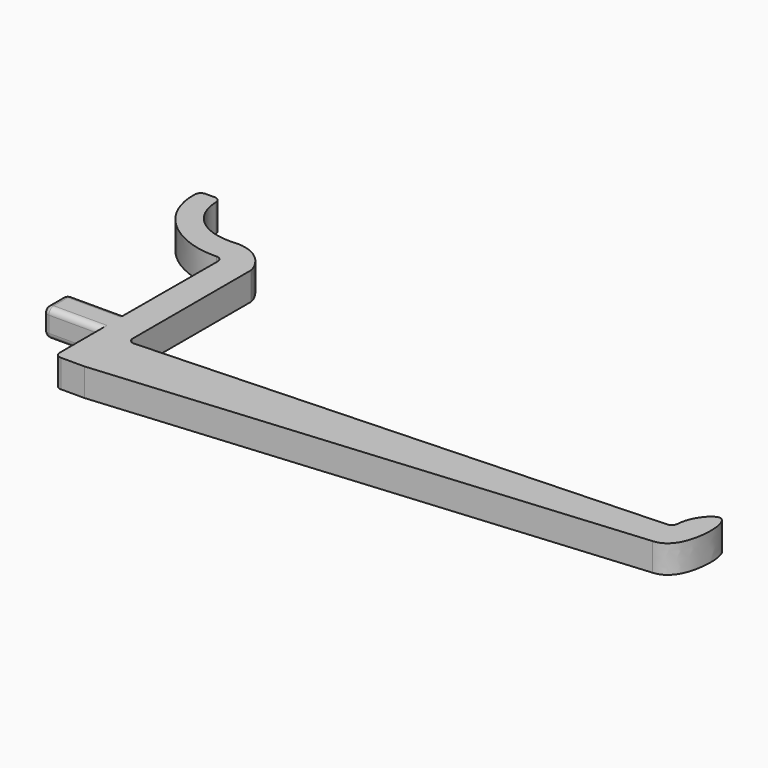
from build123d import *

# Parameters (mm, degrees)
F1_DEPTH = 4.7
F2_R     = 1


with BuildPart() as f1:
    # F0 (on Top) → F1 (new body)
    with BuildSketch(Plane.XY):
        with BuildLine():
            Line((-12.3301572212, 26.1715785798), (-15.8301572212, 26.1715785798))
            add(Edge.make_bspline(
                [(-15.8301572212, 26.1715785798), (-16.7997692679, 17.9848263993), (-8.8800950357, 12.3493980705), (-1.5833711872, 13.1881022432)],
                knots=[0, 0, 0, 0, 19.2754136163, 19.2754136163, 19.2754136163, 19.2754136163], degree=3))
            Line((-1.5833711872, 13.1881022432), (-1.6532300643, -7.3117787256))
            Line((-1.6532300643, -7.3117787256), (-11.5833711872, -7.3117787256))
            Line((-11.5833711872, -7.3117787256), (-11.5833711872, -12.3117787256))
            Line((-11.5833711872, -12.3117787256), (-1.5833711872, -12.3117787256))
            Line((-1.5833711872, -12.3117787256), (-1.5833711872, -22.3117787256))
            Line((-1.5833711872, -22.3117787256), (3.4166288128, -22.3117787256))
            Line((3.4166288128, -22.3117787256), (93.074151641, -14.4677618783))
            Line((93.074151641, -14.4677618783), (92.6383729273, -9.4867883879))
            Line((92.6383729273, -9.4867883879), (3.4166288128, -13.1708589983))
            Line((3.4166288128, -13.1708589983), (3.4166288128, 12.8291410017))
            add(Edge.make_bspline(
                [(-2.649059402, 17.6881022432), (1.8865002444, 17.5075998859), (3.3608573382, 13.5643548658), (3.4166288128, 12.8291410017)],
                knots=[0, 0, 0, 0, 7.7718773708, 7.7718773708, 7.7718773708, 7.7718773708], degree=3))
            add(Edge.make_bspline(
                [(-12.3301572212, 26.1715785798), (-12.6828875853, 21.1161755461), (-8.9998222388, 17.0332827738), (-2.649059402, 17.6881022432)],
                knots=[0, 0, 0, 0, 12.8721803023, 12.8721803023, 12.8721803023, 12.8721803023], degree=3))
        make_face()
        with BuildLine():
            add(Edge.make_bspline(
                [(92.6383729273, -9.4867883879), (92.3075102355, -6.5398698428), (96.8060362316, -0.7143486372), (97.8576879629, -9.9857558243), (95.4716324541, -14.3468420863), (93.074151641, -14.4677618783)],
                knots=[0, 0, 0, 0, 0.3422957302, 0.6624021544, 1, 1, 1, 1], degree=3))
            Line((92.6383729273, -9.4867883879), (93.074151641, -14.4677618783))
        make_face()
    extrude(amount=F1_DEPTH)

    # F2
    f2_edges = [f1.edges().sort_by_distance(p)[0] for p in [
        (-6.618301, -7.311779, 4.7),
        (-6.583371, -12.311779, 4.7),
        (-6.618301, -7.311779, 0),
        (-6.583371, -12.311779, 0),
        (-11.583371, -7.311779, 2.35),
        (-11.583371, -12.311779, 2.35),
        (-11.583371, -9.811779, 0),
        (-11.583371, -9.811779, 4.7),
        (-15.830157, 26.171579, 2.35),
        (-12.330157, 26.171579, 2.35),
        (-1.583371, 13.188102, 2.35),
        (-1.583371, -22.311779, 2.35),
        (92.638373, -9.486788, 2.35),
        (3.416629, -13.170859, 2.35),
    ]]
    fillet(f2_edges, radius=F2_R)


solid = f1.part
